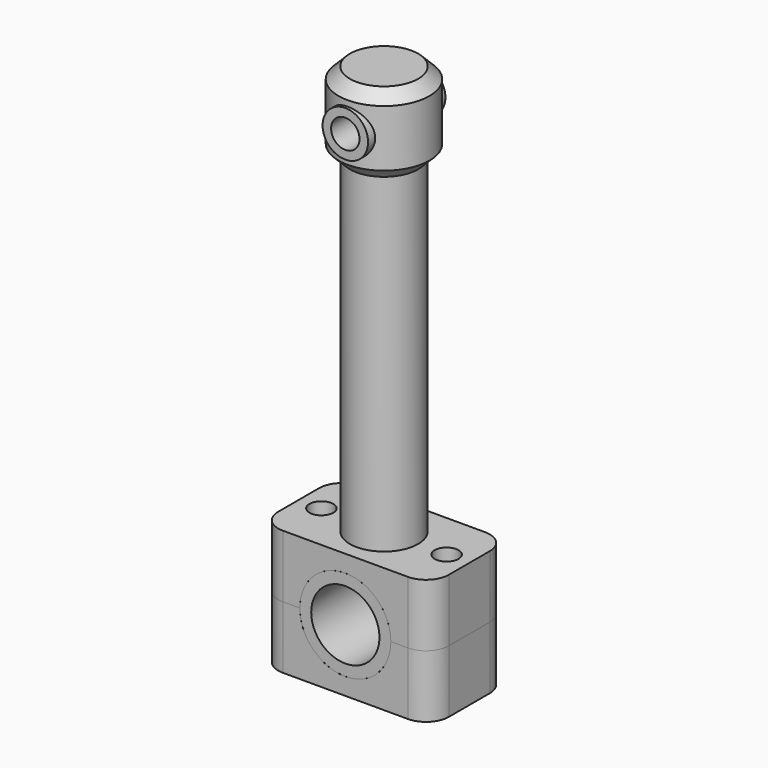
from build123d import *

# Parameters (mm, degrees)
F0_R           = 2
F1_DEPTH       = 11
F2_R           = 2
F3_DEPTH       = 11
F4_D           = 4.2
F5_R           = 6
F6_DEPTH       = 58
F7_R           = 8
F7_R_2         = 6
F8_DEPTH       = 14
F9_SIZE        = 1.99999
F11_DEPTH      = 17.001
F12_DEPTH      = 17
F13_R          = 4
F13_R_2        = 2.5
F14_DEPTH      = 8.501
F14_DEPTH_BACK = 8.501
F15_DEPTH      = 8.5


# Not quite as in the source:
# - a fillet or chamfer is up to 0.001 mm smaller than in the source, because OpenCascade refuses the exact size


with BuildPart() as f1:
    # F0 (on Top) → F1 (new body)
    with BuildSketch(Plane.XY):
        with BuildLine():
            Line((-11, -8.5), (11, -8.5))
            ThreePointArc((11, -8.5), (13.8284271247, -7.3284271247), (15, -4.5))
            Line((15, -4.5), (15, 4.5))
            ThreePointArc((15, 4.5), (13.8284271247, 7.3284271247), (11, 8.5))
            Line((11, 8.5), (-11, 8.5))
            ThreePointArc((-11, 8.5), (-13.8284271247, 7.3284271247), (-15, 4.5))
            Line((-15, 4.5), (-15, -4.5))
            ThreePointArc((-15, -4.5), (-13.8284271247, -7.3284271247), (-11, -8.5))
        make_face()
        with Locations((-11, 0)):
            Circle(F0_R, mode=Mode.SUBTRACT)
        with Locations((11, 0)):
            Circle(F0_R, mode=Mode.SUBTRACT)
    extrude(amount=F1_DEPTH)


with BuildPart() as f3:
    # F2 (on face) → F3 (new body)
    with BuildSketch(Plane.XY.offset(11)):
        with BuildLine():
            ThreePointArc((-15, -4.5), (-13.8284271247, -7.3284271247), (-11, -8.5))
            Line((-11, -8.5), (11, -8.5))
            ThreePointArc((11, -8.5), (13.8284271247, -7.3284271247), (15, -4.5))
            Line((15, -4.5), (15, 4.5))
            ThreePointArc((15, 4.5), (13.8284271247, 7.3284271247), (11, 8.5))
            Line((11, 8.5), (-11, 8.5))
            ThreePointArc((-11, 8.5), (-13.8284271247, 7.3284271247), (-15, 4.5))
            Line((-15, 4.5), (-15, -4.5))
        make_face()
        with Locations((-11, 0)):
            Circle(F2_R, mode=Mode.SUBTRACT)
        with Locations((11, 0)):
            Circle(F2_R, mode=Mode.SUBTRACT)
        with Locations((-11, 0)):
            Circle(F2_R)
        with Locations((11, 0)):
            Circle(F2_R)
    extrude(amount=F3_DEPTH)

    # F4 (through all)
    with Locations(Plane(origin=(0, 0, 11), x_dir=(1, 0, 0), z_dir=(0, 0, -1))):
        with Locations((-11, 0), (11, 0)):
            Hole(F4_D / 2)

    # F5 (on face) → F6 (join)
    with BuildSketch(Plane.XY.offset(22)):
        Circle(F5_R)
    extrude(amount=F6_DEPTH)

    # F7 (on face) → F8 (join)
    with BuildSketch(Plane.XY.offset(80)):
        Circle(F7_R)
        Circle(F7_R_2, mode=Mode.SUBTRACT)
        Circle(F7_R_2)
    extrude(amount=F8_DEPTH)

    # F9 (size 2 in the source; OpenCascade refuses exactly that, so slightly less here)
    f9_edges = [f3.edges().sort_by_distance(p)[0] for p in [
        (-8, 0, 80),
        (-8, 0, 94),
    ]]
    chamfer(f9_edges, length=F9_SIZE)


with BuildPart() as f11_tool:
    # F10 (on face) → F11 (new body, through all)
    with BuildSketch(Plane.XZ.offset(8.5)):
        with BuildLine():
            Line((-6, 11), (6, 11))
            ThreePointArc((6, 11), (0, 17), (-6, 11))
        make_face()
        with BuildLine():
            ThreePointArc((-6, 11), (0, 17), (6, 11))
            Line((6, 11), (8, 11))
            ThreePointArc((8, 11), (0, 19), (-8, 11))
            Line((-8, 11), (-6, 11))
        make_face()
        with BuildLine():
            Line((8, 11), (6, 11))
            ThreePointArc((6, 11), (0, 5), (-6, 11))
            Line((-6, 11), (-8, 11))
            ThreePointArc((-8, 11), (0, 3), (8, 11))
        make_face()
        with BuildLine():
            ThreePointArc((-6, 11), (0, 5), (6, 11))
            Line((6, 11), (-6, 11))
        make_face()
    extrude(amount=-F11_DEPTH)


with BuildPart() as f1_1:
    add(f1.part)

    # F11: cut by f11_tool
    add(f11_tool.part, mode=Mode.SUBTRACT)


with BuildPart() as f3_1:
    add(f3.part)

    # F11: cut by f11_tool
    add(f11_tool.part, mode=Mode.SUBTRACT)

    # F13 (on Front) → F14 (cut, two sides)
    with BuildSketch(Plane.XZ) as f14_sk:
        with Locations((0, 87)):
            Circle(F13_R)
        with Locations((0, 87)):
            Circle(F13_R_2, mode=Mode.SUBTRACT)
        with Locations((0, 87)):
            Circle(F13_R_2)
    extrude(amount=-F14_DEPTH, mode=Mode.SUBTRACT)
    extrude(f14_sk.sketch, amount=F14_DEPTH_BACK, mode=Mode.SUBTRACT)


with BuildPart() as f12:
    # F10 (on face) → F12 (new body)
    with BuildSketch(Plane.XZ.offset(8.5)):
        with BuildLine():
            Line((8, 11), (6, 11))
            ThreePointArc((6, 11), (0, 5), (-6, 11))
            Line((-6, 11), (-8, 11))
            ThreePointArc((-8, 11), (0, 3), (8, 11))
        make_face()
        with BuildLine():
            ThreePointArc((-6, 11), (0, 17), (6, 11))
            Line((6, 11), (8, 11))
            ThreePointArc((8, 11), (0, 19), (-8, 11))
            Line((-8, 11), (-6, 11))
        make_face()
    extrude(amount=-F12_DEPTH)


with BuildPart() as f15:
    # F13 (on Front) → F15 (new body, symmetric)
    with BuildSketch(Plane.XZ):
        with Locations((0, 87)):
            Circle(F13_R)
        with Locations((0, 87)):
            Circle(F13_R_2, mode=Mode.SUBTRACT)
    extrude(amount=F15_DEPTH, both=True)


solid = Compound([f1_1.part, f3_1.part, f12.part, f15.part])
